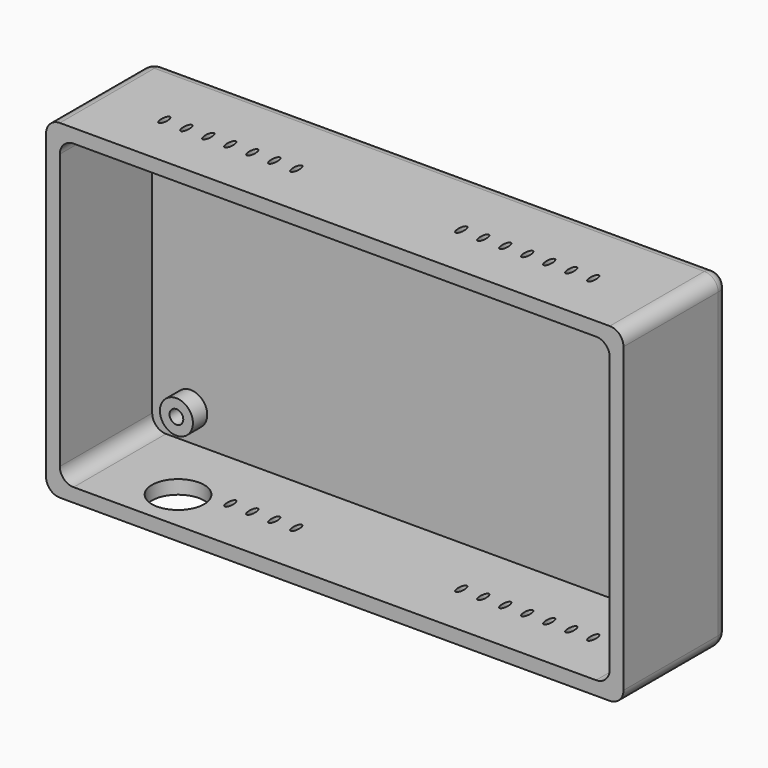
from build123d import *

# Parameters (mm, degrees)
F0_W           = 105
F0_H           = 60
F0_W_2         = 100
F0_H_2         = 55
F2_DEPTH       = 24
F1_W           = 100
F1_H           = 55
F1_R           = 3
F1_R_2         = 1.25
F3_DEPTH       = 3
F4_R           = 2.5
F5_T1_DEPTH    = 27.75
F5_S5_W        = 2.5
F5_S5_H        = 2.5
F5_T6_DEPTH    = 2.5
F5_S11_W       = 2.5
F5_S11_H       = 2.5
F5_T12_DEPTH   = 2.5
F5_S17_W       = 2.5
F5_S17_H       = 2.5
F5_T18_DEPTH   = 2.5
F5_S23_W       = 2.5
F5_S23_H       = 2.5
F5_T24_DEPTH   = 2.5
F6_R           = 2.5
F7_DEPTH       = 6.25
F9_DEPTH       = 60.001
F11_DEPTH      = 25
F11_DEPTH_BACK = 10
F10_R          = 4.75
F12_DEPTH      = 10


# Not quite as in the source:
# - a fillet or chamfer that OpenCascade refuses, or shapes differently, is made with other operations: its cross-section is extruded or revolved along the edge and cut away or added


with BuildPart() as f2:
    # F0 (on Front) → F2 (new body)
    with BuildSketch(Plane.XZ):
        Rectangle(F0_W, F0_H)
        Rectangle(F0_W_2, F0_H_2, mode=Mode.SUBTRACT)
    extrude(amount=F2_DEPTH)

    # F0 (on Front) + F1 (on face) → F3 (join)
    with BuildSketch(Plane.XZ):
        Rectangle(F0_W_2, F0_H_2)
    with BuildSketch(Plane.XZ):
        Rectangle(F1_W, F1_H)
        with Locations((-43, -22)):
            Circle(F1_R, mode=Mode.SUBTRACT)
        with Locations((43, -22)):
            Circle(F1_R, mode=Mode.SUBTRACT)
        with Locations((-43, 22)):
            Circle(F1_R, mode=Mode.SUBTRACT)
        with Locations((43, 22)):
            Circle(F1_R, mode=Mode.SUBTRACT)
        with Locations((43, 22)):
            Circle(F1_R)
        with Locations((43, 22)):
            Circle(F1_R_2, mode=Mode.SUBTRACT)
    extrude(amount=F3_DEPTH)

    # F4
    f4_edges = [f2.edges().sort_by_distance(p)[0] for p in [
        (0, 0, -30),
        (0, 0, 30),
        (-52.5, 0, 0),
        (52.5, 0, 0),
    ]]
    fillet(f4_edges, radius=F4_R)

    # F5: fillet of radius 2.5 on 4 edges, made by hand

    # F5_s2 → F5_t1 (cut)
    with BuildSketch(Plane.XZ.offset(2.5)):
        with BuildLine():
            ThreePointArc((-50, 30), (-51.767766953, 29.267766953), (-52.5, 27.5))
            Line((-52.5, 27.5), (-52.5, 30))
            Line((-52.5, 30), (-50, 30))
        make_face()
        with BuildLine():
            ThreePointArc((50, 30), (51.767766953, 29.267766953), (52.5, 27.5))
            Line((52.5, 27.5), (52.5, 30))
            Line((52.5, 30), (50, 30))
        make_face()
        with BuildLine():
            ThreePointArc((52.5, -27.5), (51.767766953, -29.267766953), (50, -30))
            Line((50, -30), (52.5, -30))
            Line((52.5, -30), (52.5, -27.5))
        make_face()
        with BuildLine():
            ThreePointArc((-52.5, -27.5), (-51.767766953, -29.267766953), (-50, -30))
            Line((-50, -30), (-52.5, -30))
            Line((-52.5, -30), (-52.5, -27.5))
        make_face()
    extrude(amount=F5_T1_DEPTH, mode=Mode.SUBTRACT)


with BuildPart() as f5_tool4:
    # F5_s5 → F5_t6 (new body)
    with BuildSketch(Plane.YZ.offset(-50)):
        with Locations((-1.25, -28.75)):
            Rectangle(F5_S5_W, F5_S5_H)
    extrude(amount=-F5_T6_DEPTH)

    # F5_s7 → F5_t8 (revolve, cut)
    with BuildSketch(Plane(origin=(-50, -2.5, -27.5), x_dir=(0, -0.7071067812, 0.7071067812), z_dir=(0, -0.7071067812, -0.7071067812))):
        with BuildLine():
            ThreePointArc((0, -2.5), (2.5, 0), (0, 2.5))
            Line((0, 2.5), (0, -2.5))
        make_face()
    revolve(axis=Axis((-50, -2.5, -27.5), (-1, 0, 0)), mode=Mode.SUBTRACT)


with BuildPart() as f2_1:
    add(f2.part)

    # F5_t3: cut F5_tool4
    add(f5_tool4.part, mode=Mode.SUBTRACT)


with BuildPart() as f5_tool10:
    # F5_s11 → F5_t12 (new body)
    with BuildSketch(Plane.YZ.offset(50)):
        with Locations((-1.25, -28.75)):
            Rectangle(F5_S11_W, F5_S11_H)
    extrude(amount=F5_T12_DEPTH)

    # F5_s13 → F5_t14 (revolve, cut)
    with BuildSketch(Plane(origin=(50, -2.5, -27.5), x_dir=(0, -0.7071067812, 0.7071067812), z_dir=(0, 0.7071067812, 0.7071067812))):
        with BuildLine():
            ThreePointArc((0, -2.5), (2.5, 0), (0, 2.5))
            Line((0, 2.5), (0, -2.5))
        make_face()
    revolve(axis=Axis((50, -2.5, -27.5), (1, 0, 0)), mode=Mode.SUBTRACT)


with BuildPart() as f2_2:
    add(f2_1.part)

    # F5_t9: cut F5_tool10
    add(f5_tool10.part, mode=Mode.SUBTRACT)


with BuildPart() as f5_tool16:
    # F5_s17 → F5_t18 (new body)
    with BuildSketch(Plane.XY.offset(27.5)):
        with Locations((51.25, -1.25)):
            Rectangle(F5_S17_W, F5_S17_H)
    extrude(amount=F5_T18_DEPTH)

    # F5_s19 → F5_t20 (revolve, cut)
    with BuildSketch(Plane(origin=(50, -2.5, 27.5), x_dir=(-0.7071067812, -0.7071067812, 0), z_dir=(-0.7071067812, 0.7071067812, 0))):
        with BuildLine():
            ThreePointArc((0, -2.5), (2.5, 0), (0, 2.5))
            Line((0, 2.5), (0, -2.5))
        make_face()
    revolve(axis=Axis((50, -2.5, 27.5), (0, 0, 1)), mode=Mode.SUBTRACT)


with BuildPart() as f2_3:
    add(f2_2.part)

    # F5_t15: cut F5_tool16
    add(f5_tool16.part, mode=Mode.SUBTRACT)


with BuildPart() as f5_tool22:
    # F5_s23 → F5_t24 (new body)
    with BuildSketch(Plane.XY.offset(27.5)):
        with Locations((-51.25, -1.25)):
            Rectangle(F5_S23_W, F5_S23_H)
    extrude(amount=F5_T24_DEPTH)

    # F5_s25 → F5_t26 (revolve, cut)
    with BuildSketch(Plane(origin=(-50, -2.5, 27.5), x_dir=(0.7071067812, -0.7071067812, 0), z_dir=(-0.7071067812, -0.7071067812, 0))):
        with BuildLine():
            ThreePointArc((0, -2.5), (2.5, 0), (0, 2.5))
            Line((0, 2.5), (0, -2.5))
        make_face()
    revolve(axis=Axis((-50, -2.5, 27.5), (0, 0, 1)), mode=Mode.SUBTRACT)


with BuildPart() as f2_4:
    add(f2_3.part)

    # F5_t21: cut F5_tool22
    add(f5_tool22.part, mode=Mode.SUBTRACT)

    # F6
    f6_edges = [f2_4.edges().sort_by_distance(p)[0] for p in [
        (-50, -13.5, -27.5),
        (-50, -13.5, 27.5),
        (50, -13.5, 27.5),
        (50, -13.5, -27.5),
    ]]
    fillet(f6_edges, radius=F6_R)

    # F1 (on face) → F7 (join)
    with BuildSketch(Plane.XZ):
        with Locations((-43, 22)):
            Circle(F1_R)
        with Locations((-43, 22)):
            Circle(F1_R_2, mode=Mode.SUBTRACT)
        with Locations((-43, -22)):
            Circle(F1_R)
        with Locations((-43, -22)):
            Circle(F1_R_2, mode=Mode.SUBTRACT)
        with Locations((43, -22)):
            Circle(F1_R)
        with Locations((43, -22)):
            Circle(F1_R_2, mode=Mode.SUBTRACT)
        with Locations((43, 22)):
            Circle(F1_R)
        with Locations((43, 22)):
            Circle(F1_R_2, mode=Mode.SUBTRACT)
    extrude(amount=F7_DEPTH)

    # F8 (on face) → F9 (cut, through all)
    with BuildSketch(Plane.XY.offset(30)):
        with BuildLine():
            add(Edge.make_bspline(
                [(14.5, -14), (14.5, -16.1650635095), (15.25, -15.0825317547), (16, -14), (15.25, -12.9174682453), (14.5, -11.8349364905), (14.5, -14)],
                knots=[4.7123889804, 4.7123889804, 4.7123889804, 6.8067840828, 6.8067840828, 8.9011791852, 8.9011791852, 10.9955742876, 10.9955742876, 10.9955742876], degree=2, weights=[1, 0.5, 1, 0.5, 1, 0.5, 1]))
        make_face()
        with BuildLine():
            add(Edge.make_bspline(
                [(18.5, -14), (18.5, -16.1650635095), (19.25, -15.0825317547), (20, -14), (19.25, -12.9174682453), (18.5, -11.8349364905), (18.5, -14)],
                knots=[4.7123889804, 4.7123889804, 4.7123889804, 6.8067840828, 6.8067840828, 8.9011791852, 8.9011791852, 10.9955742876, 10.9955742876, 10.9955742876], degree=2, weights=[1, 0.5, 1, 0.5, 1, 0.5, 1]))
        make_face()
        with BuildLine():
            add(Edge.make_bspline(
                [(22.5, -14), (22.5, -16.1650635095), (23.25, -15.0825317547), (24, -14), (23.25, -12.9174682453), (22.5, -11.8349364905), (22.5, -14)],
                knots=[4.7123889804, 4.7123889804, 4.7123889804, 6.8067840828, 6.8067840828, 8.9011791852, 8.9011791852, 10.9955742876, 10.9955742876, 10.9955742876], degree=2, weights=[1, 0.5, 1, 0.5, 1, 0.5, 1]))
        make_face()
        with BuildLine():
            add(Edge.make_bspline(
                [(26.5, -14), (26.5, -16.1650635095), (27.25, -15.0825317547), (28, -14), (27.25, -12.9174682453), (26.5, -11.8349364905), (26.5, -14)],
                knots=[4.7123889804, 4.7123889804, 4.7123889804, 6.8067840828, 6.8067840828, 8.9011791852, 8.9011791852, 10.9955742876, 10.9955742876, 10.9955742876], degree=2, weights=[1, 0.5, 1, 0.5, 1, 0.5, 1]))
        make_face()
        with BuildLine():
            add(Edge.make_bspline(
                [(30.5, -14), (30.5, -16.1650635095), (31.25, -15.0825317547), (32, -14), (31.25, -12.9174682453), (30.5, -11.8349364905), (30.5, -14)],
                knots=[4.7123889804, 4.7123889804, 4.7123889804, 6.8067840828, 6.8067840828, 8.9011791852, 8.9011791852, 10.9955742876, 10.9955742876, 10.9955742876], degree=2, weights=[1, 0.5, 1, 0.5, 1, 0.5, 1]))
        make_face()
        with BuildLine():
            add(Edge.make_bspline(
                [(34.5, -14), (34.5, -16.1650635095), (35.25, -15.0825317547), (36, -14), (35.25, -12.9174682453), (34.5, -11.8349364905), (34.5, -14)],
                knots=[4.7123889804, 4.7123889804, 4.7123889804, 6.8067840828, 6.8067840828, 8.9011791852, 8.9011791852, 10.9955742876, 10.9955742876, 10.9955742876], degree=2, weights=[1, 0.5, 1, 0.5, 1, 0.5, 1]))
        make_face()
        with BuildLine():
            add(Edge.make_bspline(
                [(38.5, -14), (38.5, -16.1650635095), (39.25, -15.0825317547), (40, -14), (39.25, -12.9174682453), (38.5, -11.8349364905), (38.5, -14)],
                knots=[4.7123889804, 4.7123889804, 4.7123889804, 6.8067840828, 6.8067840828, 8.9011791852, 8.9011791852, 10.9955742876, 10.9955742876, 10.9955742876], degree=2, weights=[1, 0.5, 1, 0.5, 1, 0.5, 1]))
        make_face()
        with BuildLine():
            add(Edge.make_bspline(
                [(-15.5, -14), (-15.5, -16.1650635095), (-14.75, -15.0825317547), (-14, -14), (-14.75, -12.9174682453), (-15.5, -11.8349364905), (-15.5, -14)],
                knots=[4.7123889804, 4.7123889804, 4.7123889804, 6.8067840828, 6.8067840828, 8.9011791852, 8.9011791852, 10.9955742876, 10.9955742876, 10.9955742876], degree=2, weights=[1, 0.5, 1, 0.5, 1, 0.5, 1]))
        make_face()
        with BuildLine():
            add(Edge.make_bspline(
                [(-19.5, -14), (-19.5, -16.1650635095), (-18.75, -15.0825317547), (-18, -14), (-18.75, -12.9174682453), (-19.5, -11.8349364905), (-19.5, -14)],
                knots=[4.7123889804, 4.7123889804, 4.7123889804, 6.8067840828, 6.8067840828, 8.9011791852, 8.9011791852, 10.9955742876, 10.9955742876, 10.9955742876], degree=2, weights=[1, 0.5, 1, 0.5, 1, 0.5, 1]))
        make_face()
        with BuildLine():
            add(Edge.make_bspline(
                [(-23.5, -14), (-23.5, -16.1650635095), (-22.75, -15.0825317547), (-22, -14), (-22.75, -12.9174682453), (-23.5, -11.8349364905), (-23.5, -14)],
                knots=[4.7123889804, 4.7123889804, 4.7123889804, 6.8067840828, 6.8067840828, 8.9011791852, 8.9011791852, 10.9955742876, 10.9955742876, 10.9955742876], degree=2, weights=[1, 0.5, 1, 0.5, 1, 0.5, 1]))
        make_face()
        with BuildLine():
            add(Edge.make_bspline(
                [(-27.5, -14), (-27.5, -16.1650635095), (-26.75, -15.0825317547), (-26, -14), (-26.75, -12.9174682453), (-27.5, -11.8349364905), (-27.5, -14)],
                knots=[4.7123889804, 4.7123889804, 4.7123889804, 6.8067840828, 6.8067840828, 8.9011791852, 8.9011791852, 10.9955742876, 10.9955742876, 10.9955742876], degree=2, weights=[1, 0.5, 1, 0.5, 1, 0.5, 1]))
        make_face()
    extrude(amount=-F9_DEPTH, mode=Mode.SUBTRACT)

    # F8 (on face) → F11 (cut, two sides)
    with BuildSketch(Plane.XY.offset(30)) as f11_sk:
        with BuildLine():
            add(Edge.make_bspline(
                [(-31.5, -14), (-31.5, -16.1650635095), (-30.75, -15.0825317547), (-30, -14), (-30.75, -12.9174682453), (-31.5, -11.8349364905), (-31.5, -14)],
                knots=[4.7123889804, 4.7123889804, 4.7123889804, 6.8067840828, 6.8067840828, 8.9011791852, 8.9011791852, 10.9955742876, 10.9955742876, 10.9955742876], degree=2, weights=[1, 0.5, 1, 0.5, 1, 0.5, 1]))
        make_face()
        with BuildLine():
            add(Edge.make_bspline(
                [(-35.5, -14), (-35.5, -16.1650635095), (-34.75, -15.0825317547), (-34, -14), (-34.75, -12.9174682453), (-35.5, -11.8349364905), (-35.5, -14)],
                knots=[4.7123889804, 4.7123889804, 4.7123889804, 6.8067840828, 6.8067840828, 8.9011791852, 8.9011791852, 10.9955742876, 10.9955742876, 10.9955742876], degree=2, weights=[1, 0.5, 1, 0.5, 1, 0.5, 1]))
        make_face()
        with BuildLine():
            add(Edge.make_bspline(
                [(-39.5, -14), (-39.5, -16.1650635095), (-38.75, -15.0825317547), (-38, -14), (-38.75, -12.9174682453), (-39.5, -11.8349364905), (-39.5, -14)],
                knots=[4.7123889804, 4.7123889804, 4.7123889804, 6.8067840828, 6.8067840828, 8.9011791852, 8.9011791852, 10.9955742876, 10.9955742876, 10.9955742876], degree=2, weights=[1, 0.5, 1, 0.5, 1, 0.5, 1]))
        make_face()
    extrude(amount=-F11_DEPTH, mode=Mode.SUBTRACT)
    extrude(f11_sk.sketch, amount=F11_DEPTH_BACK, mode=Mode.SUBTRACT)

    # F10 (on face) → F12 (cut)
    with BuildSketch(Plane(origin=(0, 0, -30), x_dir=(1, 0, 0), z_dir=(0, 0, -1))):
        with Locations((-34.5, 16.5)):
            Circle(F10_R)
    extrude(amount=-F12_DEPTH, mode=Mode.SUBTRACT)


solid = f2_4.part
